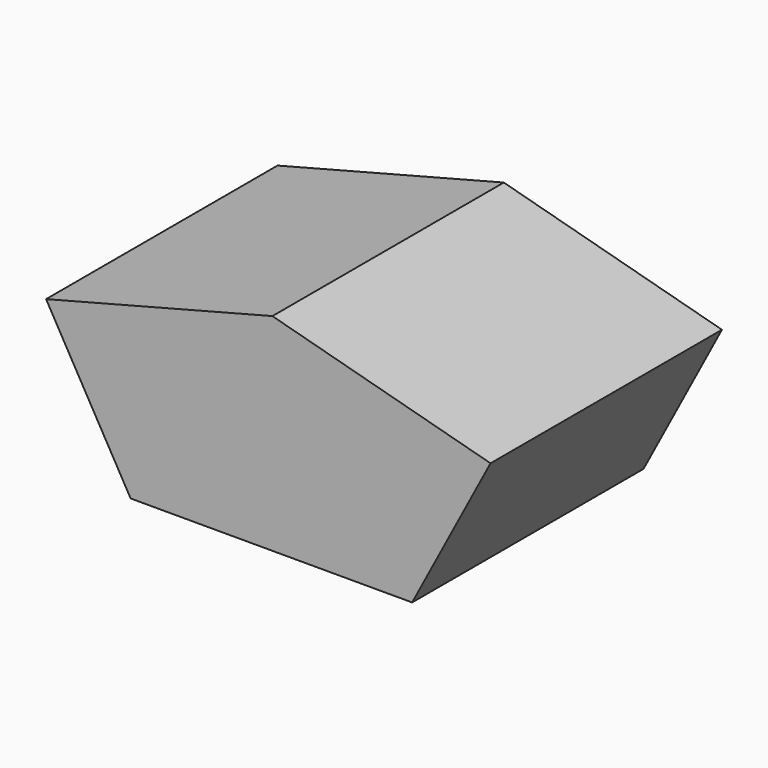
from build123d import *

# Parameters (mm, degrees)
F1_DEPTH = 63.5


# Not quite as in the source:
# - the program builds the solid bodies; features that only make, move or delete a surface that nothing else refers to are left out


with BuildPart() as f1:
    # F0 (on Front) → F1 (new body)
    with BuildSketch(Plane.XZ):
        Polygon((-31.1266705394, -32.4914753437), (30.6755751371, -32.4914753437), (47.8822439909, 0), (0, 12.877419591), (-49.6866777539, 0), align=None)
    extrude(amount=F1_DEPTH)


solid = f1.part
